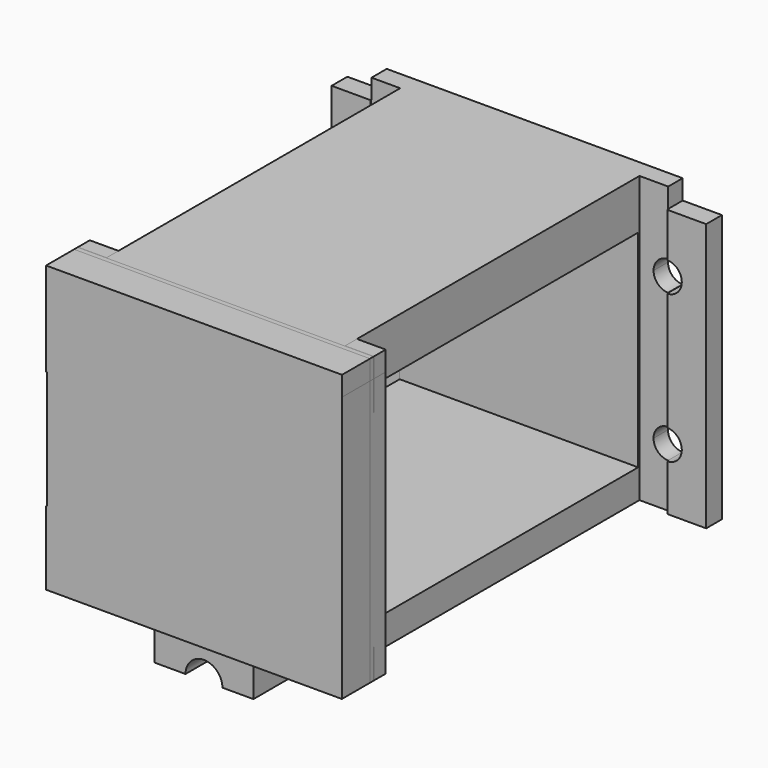
from build123d import *

# Parameters (mm, degrees)
F0_W          = 6.0148409306
F0_H          = 9.525
F0_W_2        = 5.9851590694
F0_H_2        = 6.35
F0_W_3        = 12
F0_H_3        = 2.815
F1_DEPTH      = 2.54
F2_START      = 2.54
F2_DEPTH      = 47.326875
F3_START      = 49.866875
F3_DEPTH      = 5.08
F4_START      = 47.894875
F4_DEPTH      = 2.54
F5_DEPTH      = 50.8
F6_W          = 3.7882840261
F6_H          = 47.471923288
F6_W_2        = 3.7882830948
F6_H_2        = 47.3535386845
F7_DEPTH      = 25.4
F7_DEPTH_BACK = 25.4


# Not quite as in the source:
# - a feature names something its author has since deleted; it is built from what else it names


with BuildPart() as f1:
    # F0 (on Front) → F1 (new body)
    with BuildSketch(Plane.XZ):
        with BuildLine():
            Line((4.9150146872, -18.9464773988), (-7.8555241555, -18.9464773988))
            Line((-7.8555241555, -18.9464773988), (-7.8555241555, -23.7456746399))
            Line((-7.8555241555, -23.7456746399), (-3.8515047342, -23.7456746399))
            ThreePointArc((-3.8515047342, -23.7456746399), (-1.4702547342, -21.3644246399), (0.9109952658, -23.7456746399))
            Line((0.9109952658, -23.7456746399), (4.9150146872, -23.7456746399))
            Line((4.9150146872, -23.7456746399), (4.9150146872, -18.9464773988))
        make_face()
        Polygon((-20.5555241555, 11.5334648176), (-7.4201510128, 11.5334648176), (-7.4201510128, 14.3484648176), (4.5798489872, 14.3484648176), (4.5798489872, 11.5334648176), (17.6150146872, 11.5334648176), (17.6150146872, 15.3434648176), (-20.5555241555, 15.3434648176), align=None)
        Polygon((17.6150146872, -15.1364773988), (-20.5555241555, -15.1364773988), (-20.5555241555, -18.9351737499), (-20.5555241555, -18.9464773988), (-7.8555241555, -18.9464773988), (4.9150146872, -18.9464773988), (17.6150146872, -18.9464773988), align=None)
        with BuildLine():
            Line((17.6150146872, 15.3434648176), (17.6150146872, 11.5334648176))
            Line((17.6150146872, 11.5334648176), (17.6150146872, 9.6282336699))
            ThreePointArc((17.6150146872, 9.6282336699), (18.9811953771, 9.0809544703), (19.5496899178, 7.7234648176))
            ThreePointArc((19.5496899178, 7.7234648176), (18.9917283359, 6.3764263994), (17.6446899178, 5.8184648176))
            Line((17.6446899178, 5.8184648176), (17.6446899178, -1.8015351824))
            Line((17.6446899178, -1.8015351824), (17.6446899178, -9.4215351824))
            ThreePointArc((17.6446899178, -9.4215351824), (18.9917283359, -9.9794967643), (19.5496899178, -11.3265351824))
            ThreePointArc((19.5496899178, -11.3265351824), (18.9811953771, -12.6840248351), (17.6150146872, -13.2313040347))
            Line((17.6150146872, -13.2313040347), (17.6150146872, -15.1364773988))
            Line((17.6150146872, -15.1364773988), (17.6150146872, -18.9464773988))
            Line((17.6150146872, -18.9464773988), (17.6150146872, -19.2168746144))
            Line((17.6150146872, -19.2168746144), (22.6950146872, -19.2168746144))
            Line((22.6950146872, -19.2168746144), (22.6950146872, 15.3434648176))
            Line((22.6950146872, 15.3434648176), (17.6306664944, 15.3434648176))
            Line((17.6306664944, 15.3434648176), (17.6150146872, 15.3434648176))
        make_face()
        with BuildLine():
            ThreePointArc((-20.5555241555, 5.8211025651), (-22.3603100822, 7.7234648176), (-20.5555241555, 9.62582707))
            Line((-20.5555241555, 9.62582707), (-20.5555241555, 11.5334648176))
            Line((-20.5555241555, 11.5334648176), (-20.5555241555, 15.3434648176))
            Line((-20.5555241555, 15.3434648176), (-25.6355241555, 15.3434648176))
            Line((-25.6355241555, 15.3434648176), (-25.6355241555, -18.9351737499))
            Line((-25.6355241555, -18.9351737499), (-20.5555241555, -18.9351737499))
            Line((-20.5555241555, -18.9351737499), (-20.5555241555, -15.1364773988))
            Line((-20.5555241555, -15.1364773988), (-20.5555241555, -13.2288974349))
            ThreePointArc((-20.5555241555, -13.2288974349), (-22.3603100822, -11.3265351824), (-20.5555241555, -9.42417293))
            Line((-20.5555241555, -9.42417293), (-20.5555241555, 5.8211025651))
        make_face()
        with BuildLine():
            Line((4.5798489872, 11.5334648176), (4.5798489872, 7.7234648176))
            Line((4.5798489872, 7.7234648176), (15.7396899178, 7.7234648176))
            ThreePointArc((15.7396899178, 7.7234648176), (16.2872002651, 9.0599702769), (17.6150146872, 9.6282336699))
            Line((17.6150146872, 9.6282336699), (17.6150146872, 11.5334648176))
            Line((17.6150146872, 11.5334648176), (4.5798489872, 11.5334648176))
        make_face()
        Polygon((-7.4201510128, 11.5334648176), (-7.4201510128, 7.7234648176), (-1.4053100822, 7.7234648176), (4.5798489872, 7.7234648176), (4.5798489872, 11.5334648176), align=None)
        with BuildLine():
            ThreePointArc((-20.5555241555, 9.62582707), (-19.1441813337, 9.1054801593), (-18.5503100822, 7.7234648176))
            Line((-18.5503100822, 7.7234648176), (-7.4201510128, 7.7234648176))
            Line((-7.4201510128, 7.7234648176), (-7.4201510128, 11.5334648176))
            Line((-7.4201510128, 11.5334648176), (-20.5555241555, 11.5334648176))
            Line((-20.5555241555, 11.5334648176), (-20.5555241555, 9.62582707))
        make_face()
        with BuildLine():
            Line((-1.4053100822, -11.3265351824), (-18.5503100822, -11.3265351824))
            ThreePointArc((-18.5503100822, -11.3265351824), (-19.1441813337, -12.7085505242), (-20.5555241555, -13.2288974349))
            Line((-20.5555241555, -13.2288974349), (-20.5555241555, -15.1364773988))
            Line((-20.5555241555, -15.1364773988), (17.6150146872, -15.1364773988))
            Line((17.6150146872, -15.1364773988), (17.6150146872, -13.2313040347))
            ThreePointArc((17.6150146872, -13.2313040347), (16.2872002651, -12.6630406418), (15.7396899178, -11.3265351824))
            Line((15.7396899178, -11.3265351824), (-1.4053100822, -11.3265351824))
        make_face()
        with BuildLine():
            Line((-7.4201510128, 7.7234648176), (-18.5503100822, 7.7234648176))
            ThreePointArc((-18.5503100822, 7.7234648176), (-19.1082716641, 6.3764263994), (-20.4553100822, 5.8184648176))
            Line((-20.4553100822, 5.8184648176), (-20.4553100822, -1.8015351824))
            Line((-20.4553100822, -1.8015351824), (-7.4201510128, -1.8015351824))
            Line((-7.4201510128, -1.8015351824), (-7.4201510128, 7.7234648176))
        make_face()
        with Locations((-4.4127305475, 2.9609648176)):
            Rectangle(F0_W, F0_H)
        with Locations((1.5872694525, 2.9609648176)):
            Rectangle(F0_W_2, F0_H)
        with BuildLine():
            Line((17.6150146872, -1.8015351824), (4.5798489872, -1.8015351824))
            Line((4.5798489872, -1.8015351824), (4.5798489872, -8.1515351824))
            Line((4.5798489872, -8.1515351824), (-1.4053100822, -8.1515351824))
            Line((-1.4053100822, -8.1515351824), (-1.4053100822, -11.3265351824))
            Line((-1.4053100822, -11.3265351824), (15.7396899178, -11.3265351824))
            ThreePointArc((15.7396899178, -11.3265351824), (16.2872002651, -9.9900297231), (17.6150146872, -9.4217663301))
            Line((17.6150146872, -9.4217663301), (17.6150146872, -1.8015351824))
        make_face()
        with BuildLine():
            Line((-7.4201510128, -1.8015351824), (-20.4553100822, -1.8015351824))
            Line((-20.4553100822, -1.8015351824), (-20.4553100822, -9.4215351824))
            ThreePointArc((-20.4553100822, -9.4215351824), (-19.1082716641, -9.9794967643), (-18.5503100822, -11.3265351824))
            Line((-18.5503100822, -11.3265351824), (-1.4053100822, -11.3265351824))
            Line((-1.4053100822, -11.3265351824), (-1.4053100822, -8.1515351824))
            Line((-1.4053100822, -8.1515351824), (-7.4201510128, -8.1515351824))
            Line((-7.4201510128, -8.1515351824), (-7.4201510128, -1.8015351824))
        make_face()
        with Locations((-4.4127305475, -4.9765351824)):
            Rectangle(F0_W, F0_H_2)
        with Locations((1.5872694525, -4.9765351824)):
            Rectangle(F0_W_2, F0_H_2)
        with BuildLine():
            Line((15.7396899178, 7.7234648176), (4.5798489872, 7.7234648176))
            Line((4.5798489872, 7.7234648176), (4.5798489872, -1.8015351824))
            Line((4.5798489872, -1.8015351824), (17.6150146872, -1.8015351824))
            Line((17.6150146872, -1.8015351824), (17.6150146872, 5.8186959653))
            ThreePointArc((17.6150146872, 5.8186959653), (16.2872002651, 6.3869593582), (15.7396899178, 7.7234648176))
        make_face()
        with Locations((-1.4201510128, 12.9409648176)):
            Rectangle(F0_W_3, F0_H_3)
        Polygon((-20.5555241555, 17.8834648176), (-20.5555241555, 15.3434648176), (17.6150146872, 15.3434648176), (17.6306664944, 15.3434648176), (17.6306664944, 17.8834648176), align=None)
    extrude(amount=F1_DEPTH)

    # F0 (on Front) → F2 (join)
    with BuildSketch(Plane.XZ.offset(F2_START)):
        Polygon((-20.5555241555, 11.5334648176), (-7.4201510128, 11.5334648176), (-7.4201510128, 14.3484648176), (4.5798489872, 14.3484648176), (4.5798489872, 11.5334648176), (17.6150146872, 11.5334648176), (17.6150146872, 15.3434648176), (-20.5555241555, 15.3434648176), align=None)
        Polygon((17.6150146872, -15.1364773988), (-20.5555241555, -15.1364773988), (-20.5555241555, -18.9351737499), (-20.5555241555, -18.9464773988), (-7.8555241555, -18.9464773988), (4.9150146872, -18.9464773988), (17.6150146872, -18.9464773988), align=None)
        Polygon((-20.5555241555, 17.8834648176), (-20.5555241555, 15.3434648176), (17.6150146872, 15.3434648176), (17.6306664944, 15.3434648176), (17.6306664944, 17.8834648176), align=None)
    extrude(amount=F2_DEPTH)


with BuildPart() as f3:
    # F0 (on Front) → F3 (new body)
    with BuildSketch(Plane.XZ.offset(F3_START)):
        Polygon((-20.5555241555, 11.5334648176), (-7.4201510128, 11.5334648176), (-7.4201510128, 14.3484648176), (4.5798489872, 14.3484648176), (4.5798489872, 11.5334648176), (17.6150146872, 11.5334648176), (17.6150146872, 15.3434648176), (-20.5555241555, 15.3434648176), align=None)
        Polygon((17.6150146872, -15.1364773988), (-20.5555241555, -15.1364773988), (-20.5555241555, -18.9351737499), (-20.5555241555, -18.9464773988), (-7.8555241555, -18.9464773988), (4.9150146872, -18.9464773988), (17.6150146872, -18.9464773988), align=None)
        with BuildLine():
            Line((4.5798489872, 11.5334648176), (4.5798489872, 7.7234648176))
            Line((4.5798489872, 7.7234648176), (15.7396899178, 7.7234648176))
            ThreePointArc((15.7396899178, 7.7234648176), (16.2872002651, 9.0599702769), (17.6150146872, 9.6282336699))
            Line((17.6150146872, 9.6282336699), (17.6150146872, 11.5334648176))
            Line((17.6150146872, 11.5334648176), (4.5798489872, 11.5334648176))
        make_face()
        Polygon((-7.4201510128, 11.5334648176), (-7.4201510128, 7.7234648176), (-1.4053100822, 7.7234648176), (4.5798489872, 7.7234648176), (4.5798489872, 11.5334648176), align=None)
        with BuildLine():
            ThreePointArc((-20.5555241555, 9.62582707), (-19.1441813337, 9.1054801593), (-18.5503100822, 7.7234648176))
            Line((-18.5503100822, 7.7234648176), (-7.4201510128, 7.7234648176))
            Line((-7.4201510128, 7.7234648176), (-7.4201510128, 11.5334648176))
            Line((-7.4201510128, 11.5334648176), (-20.5555241555, 11.5334648176))
            Line((-20.5555241555, 11.5334648176), (-20.5555241555, 9.62582707))
        make_face()
        with BuildLine():
            Line((-20.4553100822, 5.8184648176), (-20.4553100822, 7.7234648176))
            Line((-20.4553100822, 7.7234648176), (-18.5503100822, 7.7234648176))
            ThreePointArc((-18.5503100822, 7.7234648176), (-19.1441813337, 9.1054801593), (-20.5555241555, 9.62582707))
            Line((-20.5555241555, 9.62582707), (-20.5555241555, 5.8211025651))
            ThreePointArc((-20.5555241555, 5.8211025651), (-20.505434473, 5.8191243686), (-20.4553100822, 5.8184648176))
        make_face()
        with BuildLine():
            Line((-1.4053100822, -11.3265351824), (-18.5503100822, -11.3265351824))
            ThreePointArc((-18.5503100822, -11.3265351824), (-19.1441813337, -12.7085505242), (-20.5555241555, -13.2288974349))
            Line((-20.5555241555, -13.2288974349), (-20.5555241555, -15.1364773988))
            Line((-20.5555241555, -15.1364773988), (17.6150146872, -15.1364773988))
            Line((17.6150146872, -15.1364773988), (17.6150146872, -13.2313040347))
            ThreePointArc((17.6150146872, -13.2313040347), (16.2872002651, -12.6630406418), (15.7396899178, -11.3265351824))
            Line((15.7396899178, -11.3265351824), (-1.4053100822, -11.3265351824))
        make_face()
        with BuildLine():
            ThreePointArc((-18.5503100822, -11.3265351824), (-19.1082716641, -9.9794967643), (-20.4553100822, -9.4215351824))
            Line((-20.4553100822, -9.4215351824), (-20.4553100822, -11.3265351824))
            Line((-20.4553100822, -11.3265351824), (-18.5503100822, -11.3265351824))
        make_face()
        with BuildLine():
            Line((-20.4553100822, -11.3265351824), (-20.4553100822, -9.4215351824))
            ThreePointArc((-20.4553100822, -9.4215351824), (-20.505434473, -9.4221947335), (-20.5555241555, -9.42417293))
            Line((-20.5555241555, -9.42417293), (-20.5555241555, -13.2288974349))
            ThreePointArc((-20.5555241555, -13.2288974349), (-19.1441813337, -12.7085505242), (-18.5503100822, -11.3265351824))
            Line((-18.5503100822, -11.3265351824), (-20.4553100822, -11.3265351824))
        make_face()
        with BuildLine():
            Line((17.6150146872, -11.3265351824), (15.7396899178, -11.3265351824))
            ThreePointArc((15.7396899178, -11.3265351824), (16.2872002651, -12.6630406418), (17.6150146872, -13.2313040347))
            Line((17.6150146872, -13.2313040347), (17.6150146872, -11.3265351824))
        make_face()
        with BuildLine():
            ThreePointArc((17.6150146872, -9.4217663301), (16.2872002651, -9.9900297231), (15.7396899178, -11.3265351824))
            Line((15.7396899178, -11.3265351824), (17.6150146872, -11.3265351824))
            Line((17.6150146872, -11.3265351824), (17.6150146872, -9.4217663301))
        make_face()
        with BuildLine():
            ThreePointArc((17.6150146872, 9.6282336699), (16.2872002651, 9.0599702769), (15.7396899178, 7.7234648176))
            Line((15.7396899178, 7.7234648176), (17.6150146872, 7.7234648176))
            Line((17.6150146872, 7.7234648176), (17.6150146872, 9.6282336699))
        make_face()
        with BuildLine():
            Line((17.6150146872, 7.7234648176), (15.7396899178, 7.7234648176))
            ThreePointArc((15.7396899178, 7.7234648176), (16.2872002651, 6.3869593582), (17.6150146872, 5.8186959653))
            Line((17.6150146872, 5.8186959653), (17.6150146872, 7.7234648176))
        make_face()
        with BuildLine():
            Line((-18.5503100822, 7.7234648176), (-20.4553100822, 7.7234648176))
            Line((-20.4553100822, 7.7234648176), (-20.4553100822, 5.8184648176))
            ThreePointArc((-20.4553100822, 5.8184648176), (-19.1082716641, 6.3764263994), (-18.5503100822, 7.7234648176))
        make_face()
        with BuildLine():
            Line((15.7396899178, 7.7234648176), (4.5798489872, 7.7234648176))
            Line((4.5798489872, 7.7234648176), (4.5798489872, -1.8015351824))
            Line((4.5798489872, -1.8015351824), (17.6150146872, -1.8015351824))
            Line((17.6150146872, -1.8015351824), (17.6150146872, 5.8186959653))
            ThreePointArc((17.6150146872, 5.8186959653), (16.2872002651, 6.3869593582), (15.7396899178, 7.7234648176))
        make_face()
        with Locations((-1.4201510128, 12.9409648176)):
            Rectangle(F0_W_3, F0_H_3)
        with BuildLine():
            Line((-7.4201510128, 7.7234648176), (-18.5503100822, 7.7234648176))
            ThreePointArc((-18.5503100822, 7.7234648176), (-19.1082716641, 6.3764263994), (-20.4553100822, 5.8184648176))
            Line((-20.4553100822, 5.8184648176), (-20.4553100822, -1.8015351824))
            Line((-20.4553100822, -1.8015351824), (-7.4201510128, -1.8015351824))
            Line((-7.4201510128, -1.8015351824), (-7.4201510128, 7.7234648176))
        make_face()
        with Locations((-4.4127305475, 2.9609648176)):
            Rectangle(F0_W, F0_H)
        with BuildLine():
            Line((17.6150146872, -1.8015351824), (4.5798489872, -1.8015351824))
            Line((4.5798489872, -1.8015351824), (4.5798489872, -8.1515351824))
            Line((4.5798489872, -8.1515351824), (-1.4053100822, -8.1515351824))
            Line((-1.4053100822, -8.1515351824), (-1.4053100822, -11.3265351824))
            Line((-1.4053100822, -11.3265351824), (15.7396899178, -11.3265351824))
            ThreePointArc((15.7396899178, -11.3265351824), (16.2872002651, -9.9900297231), (17.6150146872, -9.4217663301))
            Line((17.6150146872, -9.4217663301), (17.6150146872, -1.8015351824))
        make_face()
        with BuildLine():
            Line((-7.4201510128, -1.8015351824), (-20.4553100822, -1.8015351824))
            Line((-20.4553100822, -1.8015351824), (-20.4553100822, -9.4215351824))
            ThreePointArc((-20.4553100822, -9.4215351824), (-19.1082716641, -9.9794967643), (-18.5503100822, -11.3265351824))
            Line((-18.5503100822, -11.3265351824), (-1.4053100822, -11.3265351824))
            Line((-1.4053100822, -11.3265351824), (-1.4053100822, -8.1515351824))
            Line((-1.4053100822, -8.1515351824), (-7.4201510128, -8.1515351824))
            Line((-7.4201510128, -8.1515351824), (-7.4201510128, -1.8015351824))
        make_face()
        with Locations((-4.4127305475, -4.9765351824)):
            Rectangle(F0_W, F0_H_2)
        with Locations((1.5872694525, -4.9765351824)):
            Rectangle(F0_W_2, F0_H_2)
        with Locations((1.5872694525, 2.9609648176)):
            Rectangle(F0_W_2, F0_H)
        Polygon((-20.5555241555, 17.8834648176), (-20.5555241555, 15.3434648176), (17.6150146872, 15.3434648176), (17.6306664944, 15.3434648176), (17.6306664944, 17.8834648176), align=None)
    extrude(amount=F3_DEPTH)


with BuildPart() as f4:
    # F0 (on Front) → F4 (new body)
    with BuildSketch(Plane.XZ.offset(F4_START)):
        with BuildLine():
            Line((-18.5503100822, 7.7234648176), (-20.4553100822, 7.7234648176))
            Line((-20.4553100822, 7.7234648176), (-20.4553100822, 5.8184648176))
            ThreePointArc((-20.4553100822, 5.8184648176), (-19.1082716641, 6.3764263994), (-18.5503100822, 7.7234648176))
        make_face()
        with BuildLine():
            ThreePointArc((-18.5503100822, -11.3265351824), (-19.1082716641, -9.9794967643), (-20.4553100822, -9.4215351824))
            Line((-20.4553100822, -9.4215351824), (-20.4553100822, -11.3265351824))
            Line((-20.4553100822, -11.3265351824), (-18.5503100822, -11.3265351824))
        make_face()
        with BuildLine():
            ThreePointArc((17.6150146872, -9.4217663301), (16.2872002651, -9.9900297231), (15.7396899178, -11.3265351824))
            Line((15.7396899178, -11.3265351824), (17.6150146872, -11.3265351824))
            Line((17.6150146872, -11.3265351824), (17.6150146872, -9.4217663301))
        make_face()
        with BuildLine():
            Line((17.6150146872, 7.7234648176), (15.7396899178, 7.7234648176))
            ThreePointArc((15.7396899178, 7.7234648176), (16.2872002651, 6.3869593582), (17.6150146872, 5.8186959653))
            Line((17.6150146872, 5.8186959653), (17.6150146872, 7.7234648176))
        make_face()
        with BuildLine():
            Line((-7.4201510128, 7.7234648176), (-18.5503100822, 7.7234648176))
            ThreePointArc((-18.5503100822, 7.7234648176), (-19.1082716641, 6.3764263994), (-20.4553100822, 5.8184648176))
            Line((-20.4553100822, 5.8184648176), (-20.4553100822, -1.8015351824))
            Line((-20.4553100822, -1.8015351824), (-7.4201510128, -1.8015351824))
            Line((-7.4201510128, -1.8015351824), (-7.4201510128, 7.7234648176))
        make_face()
        with BuildLine():
            Line((4.5798489872, 11.5334648176), (4.5798489872, 7.7234648176))
            Line((4.5798489872, 7.7234648176), (15.7396899178, 7.7234648176))
            ThreePointArc((15.7396899178, 7.7234648176), (16.2872002651, 9.0599702769), (17.6150146872, 9.6282336699))
            Line((17.6150146872, 9.6282336699), (17.6150146872, 11.5334648176))
            Line((17.6150146872, 11.5334648176), (4.5798489872, 11.5334648176))
        make_face()
        with BuildLine():
            Line((15.7396899178, 7.7234648176), (4.5798489872, 7.7234648176))
            Line((4.5798489872, 7.7234648176), (4.5798489872, -1.8015351824))
            Line((4.5798489872, -1.8015351824), (17.6150146872, -1.8015351824))
            Line((17.6150146872, -1.8015351824), (17.6150146872, 5.8186959653))
            ThreePointArc((17.6150146872, 5.8186959653), (16.2872002651, 6.3869593582), (15.7396899178, 7.7234648176))
        make_face()
        with BuildLine():
            Line((17.6150146872, -1.8015351824), (4.5798489872, -1.8015351824))
            Line((4.5798489872, -1.8015351824), (4.5798489872, -8.1515351824))
            Line((4.5798489872, -8.1515351824), (-1.4053100822, -8.1515351824))
            Line((-1.4053100822, -8.1515351824), (-1.4053100822, -11.3265351824))
            Line((-1.4053100822, -11.3265351824), (15.7396899178, -11.3265351824))
            ThreePointArc((15.7396899178, -11.3265351824), (16.2872002651, -9.9900297231), (17.6150146872, -9.4217663301))
            Line((17.6150146872, -9.4217663301), (17.6150146872, -1.8015351824))
        make_face()
        with BuildLine():
            Line((-7.4201510128, -1.8015351824), (-20.4553100822, -1.8015351824))
            Line((-20.4553100822, -1.8015351824), (-20.4553100822, -9.4215351824))
            ThreePointArc((-20.4553100822, -9.4215351824), (-19.1082716641, -9.9794967643), (-18.5503100822, -11.3265351824))
            Line((-18.5503100822, -11.3265351824), (-1.4053100822, -11.3265351824))
            Line((-1.4053100822, -11.3265351824), (-1.4053100822, -8.1515351824))
            Line((-1.4053100822, -8.1515351824), (-7.4201510128, -8.1515351824))
            Line((-7.4201510128, -8.1515351824), (-7.4201510128, -1.8015351824))
        make_face()
        Polygon((-20.5555241555, 11.5334648176), (-7.4201510128, 11.5334648176), (-7.4201510128, 14.3484648176), (4.5798489872, 14.3484648176), (4.5798489872, 11.5334648176), (17.6150146872, 11.5334648176), (17.6150146872, 15.3434648176), (-20.5555241555, 15.3434648176), align=None)
        Polygon((-20.5555241555, 17.8834648176), (-20.5555241555, 15.3434648176), (17.6150146872, 15.3434648176), (17.6306664944, 15.3434648176), (17.6306664944, 17.8834648176), align=None)
        with BuildLine():
            ThreePointArc((-20.5555241555, 9.62582707), (-19.1441813337, 9.1054801593), (-18.5503100822, 7.7234648176))
            Line((-18.5503100822, 7.7234648176), (-7.4201510128, 7.7234648176))
            Line((-7.4201510128, 7.7234648176), (-7.4201510128, 11.5334648176))
            Line((-7.4201510128, 11.5334648176), (-20.5555241555, 11.5334648176))
            Line((-20.5555241555, 11.5334648176), (-20.5555241555, 9.62582707))
        make_face()
        with BuildLine():
            Line((-20.4553100822, 5.8184648176), (-20.4553100822, 7.7234648176))
            Line((-20.4553100822, 7.7234648176), (-18.5503100822, 7.7234648176))
            ThreePointArc((-18.5503100822, 7.7234648176), (-19.1441813337, 9.1054801593), (-20.5555241555, 9.62582707))
            Line((-20.5555241555, 9.62582707), (-20.5555241555, 5.8211025651))
            ThreePointArc((-20.5555241555, 5.8211025651), (-20.505434473, 5.8191243686), (-20.4553100822, 5.8184648176))
        make_face()
        with BuildLine():
            ThreePointArc((17.6150146872, 9.6282336699), (16.2872002651, 9.0599702769), (15.7396899178, 7.7234648176))
            Line((15.7396899178, 7.7234648176), (17.6150146872, 7.7234648176))
            Line((17.6150146872, 7.7234648176), (17.6150146872, 9.6282336699))
        make_face()
        Polygon((17.6150146872, -15.1364773988), (-20.5555241555, -15.1364773988), (-20.5555241555, -18.9351737499), (-20.5555241555, -18.9464773988), (-7.8555241555, -18.9464773988), (4.9150146872, -18.9464773988), (17.6150146872, -18.9464773988), align=None)
        with BuildLine():
            Line((-1.4053100822, -11.3265351824), (-18.5503100822, -11.3265351824))
            ThreePointArc((-18.5503100822, -11.3265351824), (-19.1441813337, -12.7085505242), (-20.5555241555, -13.2288974349))
            Line((-20.5555241555, -13.2288974349), (-20.5555241555, -15.1364773988))
            Line((-20.5555241555, -15.1364773988), (17.6150146872, -15.1364773988))
            Line((17.6150146872, -15.1364773988), (17.6150146872, -13.2313040347))
            ThreePointArc((17.6150146872, -13.2313040347), (16.2872002651, -12.6630406418), (15.7396899178, -11.3265351824))
            Line((15.7396899178, -11.3265351824), (-1.4053100822, -11.3265351824))
        make_face()
        with BuildLine():
            Line((17.6150146872, -11.3265351824), (15.7396899178, -11.3265351824))
            ThreePointArc((15.7396899178, -11.3265351824), (16.2872002651, -12.6630406418), (17.6150146872, -13.2313040347))
            Line((17.6150146872, -13.2313040347), (17.6150146872, -11.3265351824))
        make_face()
        with BuildLine():
            Line((-20.4553100822, -11.3265351824), (-20.4553100822, -9.4215351824))
            ThreePointArc((-20.4553100822, -9.4215351824), (-20.505434473, -9.4221947335), (-20.5555241555, -9.42417293))
            Line((-20.5555241555, -9.42417293), (-20.5555241555, -13.2288974349))
            ThreePointArc((-20.5555241555, -13.2288974349), (-19.1441813337, -12.7085505242), (-18.5503100822, -11.3265351824))
            Line((-18.5503100822, -11.3265351824), (-20.4553100822, -11.3265351824))
        make_face()
        with BuildLine():
            Line((4.9150146872, -18.9464773988), (-7.8555241555, -18.9464773988))
            Line((-7.8555241555, -18.9464773988), (-7.8555241555, -23.7456746399))
            Line((-7.8555241555, -23.7456746399), (-3.8515047342, -23.7456746399))
            ThreePointArc((-3.8515047342, -23.7456746399), (-1.4702547342, -21.3644246399), (0.9109952658, -23.7456746399))
            Line((0.9109952658, -23.7456746399), (4.9150146872, -23.7456746399))
            Line((4.9150146872, -23.7456746399), (4.9150146872, -18.9464773988))
        make_face()
    extrude(amount=F4_DEPTH)


with BuildPart() as f5:
    # F5 (new): a face of the model
    f5_faces = [f1.part.faces().sort_by_distance(p)[0] for p in [
        (-1.4702547342, -2.54, -21.1098954037),
    ]]
    extrude(f5_faces, amount=F5_DEPTH)


with BuildPart() as f1_1:
    add(f1.part)

    # F6 (on Top) → F7 (cut, two sides)
    with BuildSketch(Plane.XY) as f7_sk:
        with Locations((15.8150778152, -26.0699142236)):
            Rectangle(F6_W, F6_H)
        with Locations((-18.7530079857, -26.1291065253)):
            Rectangle(F6_W_2, F6_H_2)
    extrude(amount=-F7_DEPTH, mode=Mode.SUBTRACT)
    extrude(f7_sk.sketch, amount=F7_DEPTH_BACK, mode=Mode.SUBTRACT)


solid = Compound([f3.part, f4.part, f5.part, f1_1.part])
